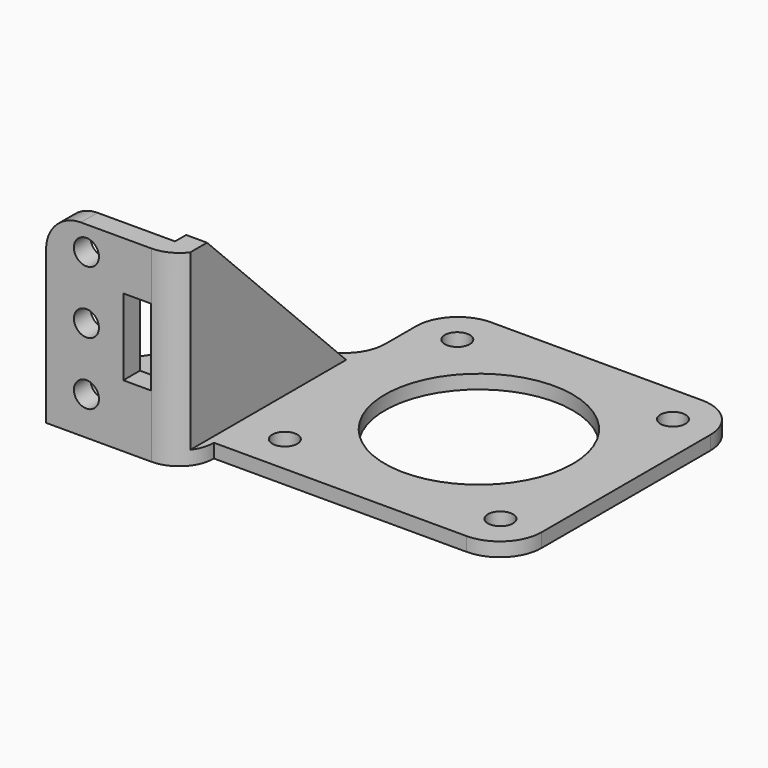
from build123d import *

# Parameters (mm, degrees)
F0_R         = 1.8
F0_R_2       = 13.5
F0_W         = 20.1372796029
F0_H         = 5
F1_DEPTH     = 2
F2_W         = 3
F2_H         = 30
F3_DEPTH     = 27
F4_W         = 16.1372796029
F4_H         = 3
F5_DEPTH     = 25
F6_R         = 1.8
F6_W         = 4
F6_H         = 11
F7_DEPTH     = 25
F8_SIZE      = 25
F9_SIZE      = 14
F10_R        = 4.99999
F11_T1_DEPTH = 2
F11_T3_DEPTH = 32


# Not quite as in the source:
# - a fillet or chamfer that OpenCascade refuses, or shapes differently, is made with other operations: its cross-section is extruded or revolved along the edge and cut away or added
# - a fillet or chamfer is up to 0.001 mm smaller than in the source, because OpenCascade refuses the exact size


with BuildPart() as f1:
    # F0 (on Top) → F1 (new body)
    with BuildSketch(Plane.XY):
        Polygon((21.15, -21.15), (21.15, 21.15), (-21.15, 21.15), (-21.15, 3.85), (-21.15, -21.15), align=None)
        with Locations((-15.5, -15.5)):
            Circle(F0_R, mode=Mode.SUBTRACT)
        with Locations((15.5, -15.5)):
            Circle(F0_R, mode=Mode.SUBTRACT)
        with Locations((-15.5, 15.5)):
            Circle(F0_R, mode=Mode.SUBTRACT)
        Circle(F0_R_2, mode=Mode.SUBTRACT)
        with Locations((15.5, 15.5)):
            Circle(F0_R, mode=Mode.SUBTRACT)
        Polygon((-21.15, -21.15), (-21.15, 3.85), (-41.3, 3.85), (-41.3, -21.15), (-21.1627203971, -21.15), align=None)
        with Locations((-31.2313601986, -23.65)):
            Rectangle(F0_W, F0_H)
    extrude(amount=F1_DEPTH)

    # F2 (on Top) → F3 (join)
    with BuildSketch(Plane.XY):
        with Locations((-23.6627203971, -11.15)):
            Rectangle(F2_W, F2_H)
    extrude(amount=F3_DEPTH)

    # F4 (on face) → F5 (join)
    with BuildSketch(Plane.XY.offset(2)):
        with Locations((-33.2313601986, -24.65)):
            Rectangle(F4_W, F4_H)
    extrude(amount=F5_DEPTH)

    # F6 (on face) → F7 (cut)
    with BuildSketch(Plane(origin=(0, -23.15, 0), x_dir=(-1, 0, 0), z_dir=(0, 1, 0))):
        with Locations((35.5, 14.5)):
            Circle(F6_R)
        with Locations((35.5, 5.5)):
            Circle(F6_R)
        with Locations((35.5, 23.5)):
            Circle(F6_R)
        with Locations((28.2, 14.5)):
            Rectangle(F6_W, F6_H)
    extrude(amount=-F7_DEPTH, mode=Mode.SUBTRACT)

    # F8
    f8_edges = [f1.edges().sort_by_distance(p)[0] for p in [
        (-23.66272, 3.85, 27),
    ]]
    chamfer(f8_edges, length=F8_SIZE)

    # F9
    f9_edges = [f1.edges().sort_by_distance(p)[0] for p in [
        (-41.3, 3.85, 1),
    ]]
    chamfer(f9_edges, length=F9_SIZE)

    # F10 (radius 5 in the source; OpenCascade refuses exactly that, so slightly less here)
    f10_edges = [f1.edges().sort_by_distance(p)[0] for p in [
        (-41.3, -10.15, 1),
        (-27.3, 3.85, 1),
        (-21.16272, -26.15, 1),
        (-41.3, -24.65, 27),
    ]]
    fillet(f10_edges, radius=F10_R)

    # F11: fillet of radius 6 on 4 edges, made by hand

    # F11_s2 → F11_t1 (join)
    with BuildSketch(Plane.XY):
        with BuildLine():
            ThreePointArc((-26.1021461366, 3.7731598692), (-22.5517871308, 5.8265464621), (-21.15, 9.6809515277))
            Line((-21.15, 9.6809515277), (-20.55, 9.6809515277))
            Line((-20.55, 9.6809515277), (-20.55, 3.85))
            Line((-20.55, 3.85), (-21.15, 3.25))
            ThreePointArc((-21.15, 3.25), (-25.2289363303, 3.25), (-25.9973607503, 3.1823807033))
            Line((-25.9973607503, 3.1823807033), (-26.1021461366, 3.7731598692))
        make_face()
    extrude(amount=F11_T1_DEPTH)

    # F11_s4 → F11_t3 (cut)
    with BuildSketch(Plane.XY.offset(-15)):
        with BuildLine():
            ThreePointArc((21.15, -15.15), (19.3926406871, -19.3926406871), (15.15, -21.15))
            Line((15.15, -21.15), (21.15, -21.15))
            Line((21.15, -21.15), (21.15, -15.15))
        make_face()
        with BuildLine():
            ThreePointArc((15.15, 21.15), (19.3926406871, 19.3926406871), (21.15, 15.15))
            Line((21.15, 15.15), (21.15, 21.15))
            Line((21.15, 21.15), (15.15, 21.15))
        make_face()
        with BuildLine():
            ThreePointArc((-21.15, 15.15), (-19.3926406871, 19.3926406871), (-15.15, 21.15))
            Line((-15.15, 21.15), (-21.15, 21.15))
            Line((-21.15, 21.15), (-21.15, 15.15))
        make_face()
    extrude(amount=F11_T3_DEPTH, mode=Mode.SUBTRACT)


solid = f1.part
